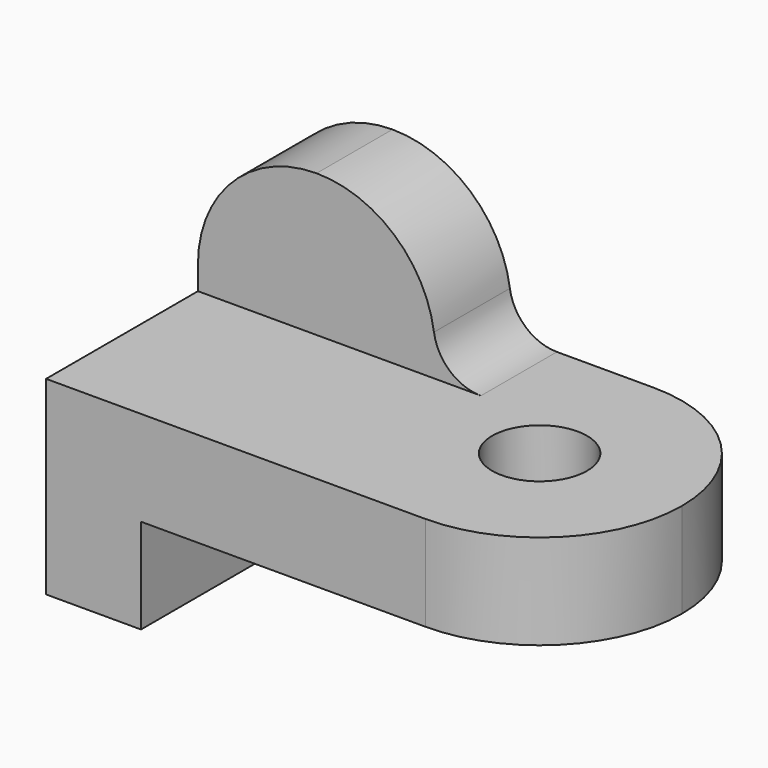
from build123d import *

# Parameters (mm, degrees)
F0_W         = 139.7
F0_H         = 88.9
F1_DEPTH     = 76.2
F2_W         = 76.2
F2_H         = 38.1
F3_DEPTH     = 76.2
F4_W         = 114.3
F4_H         = 25.4
F5_DEPTH     = 76.2
F6_W         = 63.5
F6_H         = 50.8
F7_DEPTH     = 38.1
F8_R         = 31.74999
F9_R         = 38.09999
F10_T1_DEPTH = 25.4
F11_R        = 12.7
F12_DEPTH    = 25.4


# Not quite as in the source:
# - a fillet or chamfer that OpenCascade refuses, or shapes differently, is made with other operations: its cross-section is extruded or revolved along the edge and cut away or added
# - a fillet or chamfer is up to 0.001 mm smaller than in the source, because OpenCascade refuses the exact size


with BuildPart() as f1:
    # F0 (on Front) → F1 (new body)
    with BuildSketch(Plane.XZ):
        Rectangle(F0_W, F0_H)
    extrude(amount=F1_DEPTH)

    # F2 (on face) → F3 (cut)
    with BuildSketch(Plane.XZ.offset(76.2)):
        with Locations((31.75, 25.4)):
            Rectangle(F2_W, F2_H)
    extrude(amount=-F3_DEPTH, mode=Mode.SUBTRACT)

    # F4 (on face) → F5 (cut)
    with BuildSketch(Plane.XZ.offset(76.2)):
        with Locations((12.7, -31.75)):
            Rectangle(F4_W, F4_H)
    extrude(amount=-F5_DEPTH, mode=Mode.SUBTRACT)

    # F6 (on face) → F7 (cut)
    with BuildSketch(Plane.XY.offset(44.45)):
        with Locations((-38.1, -50.8)):
            Rectangle(F6_W, F6_H)
    extrude(amount=-F7_DEPTH, mode=Mode.SUBTRACT)

    # F8 (radius 31.75 in the source; OpenCascade refuses exactly that, so slightly less here)
    f8_edges = [f1.edges().sort_by_distance(p)[0] for p in [
        (-69.85, -12.7, 44.45),
        (-6.35, -12.7, 44.45),
    ]]
    fillet(f8_edges, radius=F8_R)

    # F9 (radius 38.1 in the source; OpenCascade refuses exactly that, so slightly less here)
    f9_edges = [f1.edges().sort_by_distance(p)[0] for p in [
        (69.85, -76.2, -6.35),
        (69.85, 0, -6.35),
    ]]
    fillet(f9_edges, radius=F9_R)

    # F10: fillet of radius 12.7 on 1 edges, made by hand

    # F10_s2 → F10_t1 (join)
    with BuildSketch(Plane.XZ):
        with BuildLine():
            ThreePointArc((5.894091852, 6.35), (-2.4200107012, 9.4497031955), (-6.6756486478, 17.2357167347))
            Line((-6.6756486478, 17.2357167347), (-7.9326226978, 17.0542884082))
            ThreePointArc((-7.9326226978, 17.0542884082), (-7.62, 12.70001), (-7.62, 6.35))
            Line((-7.62, 6.35), (-6.35, 5.08))
            Line((-6.35, 5.08), (5.894091852, 5.08))
            Line((5.894091852, 5.08), (5.894091852, 6.35))
        make_face()
    extrude(amount=F10_T1_DEPTH)

    # F11 (on face) → F12 (cut)
    with BuildSketch(Plane.XY.offset(6.35)):
        with Locations((31.75, -38.1)):
            Circle(F11_R)
    extrude(amount=-F12_DEPTH, mode=Mode.SUBTRACT)


solid = f1.part
